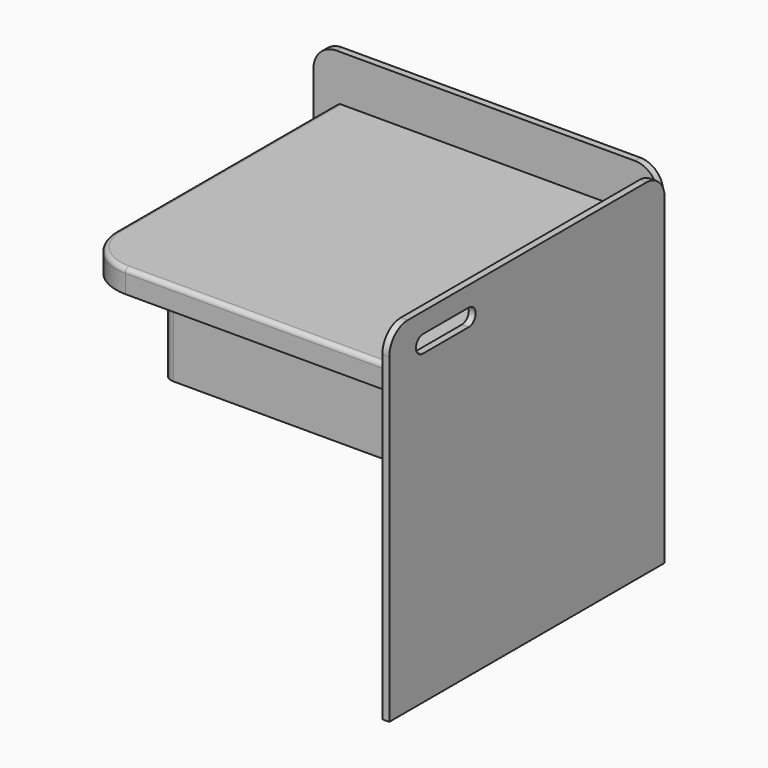
from build123d import *

# Parameters (mm, degrees)
F0_W      = 38.1
F0_H      = 38.1
F2_DEPTH  = 0.762
F1_W      = 38.1
F1_H      = 38.1
F3_DEPTH  = 0.762
F4_W      = 35.56
F4_H      = 35.56
F5_DEPTH  = 17.78
F8_W      = 30.48
F8_H      = 30.48
F9_DEPTH  = 10.16
F7_W      = 35.56
F7_H      = 35.56
F10_DEPTH = 2.54
F11_W     = 30.48
F11_H     = 12.7
F12_DEPTH = 1.27
F13_R     = 1.27
F14_DEPTH = 1.27
F16_R     = 1.27
F17_DEPTH = 2.54
F15_W     = 25.4
F15_H     = 7.62
F18_DEPTH = 1.27
F19_R     = 2.54
F19_2_R   = 2.54
F20_R     = 5.08
F21_R     = 1.27
F21_2_R   = 1.27
F23_DEPTH = 12.7
F24_DEPTH = 0.762
F26_W     = 38.1
F26_H     = 38.1
F27_DEPTH = 0.762
F29_DEPTH = 12.7
F30_R     = 2.54
F30_2_R   = 2.54
F31_T     = 1.27
F33_DEPTH = 25.4
F34_R     = 0.508
F35_R     = 0.508
F36_R     = 0.508
F37_R     = 2.54
F38_R     = 1.27


# Not quite as in the source:
# - a shell that OpenCascade refuses in one call is made with other operations: the cavity is built on its own and cut out
# - a feature names something its author has since deleted; it is built from what else it names


with BuildPart() as f2:
    # F0 (on Right) → F2 (new body)
    with BuildSketch(Plane.YZ):
        with Locations((-19.05, 19.05)):
            Rectangle(F0_W, F0_H)
    extrude(amount=-F2_DEPTH)

    # F19
    f19_edges = [f2.edges().sort_by_distance(p)[0] for p in [
        (-0.381, -38.1, 38.1),
        (-0.381, 0, 38.1),
    ]]
    fillet(f19_edges, radius=F19_R)

    # F22 (on face) → F23 (cut)
    with BuildSketch(Plane.YZ):
        with BuildLine():
            ThreePointArc((35.283215344, 34.4806989491), (34.330715344, 35.4331989491), (33.378215344, 34.4806989491))
            Line((33.378215344, 34.4806989491), (33.378215344, 28.1306989491))
            ThreePointArc((33.378215344, 28.1306989491), (34.330715344, 27.1781989491), (35.283215344, 28.1306989491))
            Line((35.283215344, 28.1306989491), (35.283215344, 34.4806989491))
        make_face()
    extrude(amount=-F23_DEPTH, mode=Mode.SUBTRACT)

    # F32 (on face) → F33 (cut)
    with BuildSketch(Plane(origin=(-0.762, 0, 0), x_dir=(0, -1, 0), z_dir=(-1, 0, 0))):
        with BuildLine():
            ThreePointArc((35.2714537645, 33.5571871057), (34.3189537645, 34.5096871057), (33.3664537645, 33.5571871057))
            Line((33.3664537645, 33.5571871057), (33.3664537645, 27.2071871057))
            ThreePointArc((33.3664537645, 27.2071871057), (34.3189537645, 26.2546871057), (35.2714537645, 27.2071871057))
            Line((35.2714537645, 27.2071871057), (35.2714537645, 33.5571871057))
        make_face()
    extrude(amount=-F33_DEPTH, mode=Mode.SUBTRACT)


with BuildPart() as f3:
    # F1 (on Front) → F3 (new body)
    with BuildSketch(Plane.XZ):
        with Locations((19.05, 19.05)):
            Rectangle(F1_W, F1_H)
    extrude(amount=F3_DEPTH)

    # F19#2
    f19_2_edges = [f3.edges().sort_by_distance(p)[0] for p in [
        (0, -0.381, 38.1),
    ]]
    fillet(f19_2_edges, radius=F19_2_R)


with BuildPart() as f5:
    # F4 (on Top) → F5 (new body)
    with BuildSketch(Plane.XY):
        with Locations((17.78, -18.5785688174)):
            Rectangle(F4_W, F4_H)
    extrude(amount=F5_DEPTH)

    # F21
    f21_edges = [f5.edges().sort_by_distance(p)[0] for p in [
        (35.56, -18.578569, 17.78),
    ]]
    fillet(f21_edges, radius=F21_R)


with BuildPart() as f9:
    # F8 (on offset) → F9 (new body)
    with BuildSketch(Plane.XY.offset(30.48)):
        with Locations((60.96, -16.002)):
            Rectangle(F8_W, F8_H)
    extrude(amount=-F9_DEPTH)

    # F21#2
    f21_2_edges = [f9.edges().sort_by_distance(p)[0] for p in [
        (45.72, -31.242, 25.4),
    ]]
    fillet(f21_2_edges, radius=F21_2_R)

    # F31: shell of thickness 1.27, made by hand


with BuildPart() as f10:
    # F7 (on offset) → F10 (new body)
    with BuildSketch(Plane.XY.offset(30.48)):
        with Locations((58.42, -18.542)):
            Rectangle(F7_W, F7_H)
    extrude(amount=F10_DEPTH)

    # F20
    f20_edges = [f10.edges().sort_by_distance(p)[0] for p in [
        (40.64, -36.322, 31.75),
    ]]
    fillet(f20_edges, radius=F20_R)

    # F34
    f34_edges = [f10.edges().sort_by_distance(p)[0] for p in [
        (40.64, -16.002, 33.02),
    ]]
    fillet(f34_edges, radius=F34_R)


with BuildPart() as f12:
    # F11 (on face) → F12 (new body)
    with BuildSketch(Plane.XZ.offset(36.3585688174)):
        with Locations((18.542, 8.89)):
            Rectangle(F11_W, F11_H)
    extrude(amount=F12_DEPTH)

    # F37
    f37_edges = [f12.edges().sort_by_distance(p)[0] for p in [
        (3.302, -36.993569, 15.24),
        (3.302, -36.993569, 2.54),
        (33.782, -36.993569, 2.54),
        (33.782, -36.993569, 15.24),
    ]]
    fillet(f37_edges, radius=F37_R)


with BuildPart() as f14:
    # F13 (on face) → F14 (new body)
    with BuildSketch(Plane.XZ.offset(37.6285688174)):
        with Locations((18.542, 8.89)):
            Circle(F13_R)
    extrude(amount=F14_DEPTH)

    # F35
    f35_edges = [f14.edges().sort_by_distance(p)[0] for p in [
        (17.272, -38.898569, 8.89),
    ]]
    fillet(f35_edges, radius=F35_R)


with BuildPart() as f17:
    # F16 (on face) → F17 (new body)
    with BuildSketch(Plane(origin=(45.72, 0, 0), x_dir=(0, -1, 0), z_dir=(-1, 0, 0))):
        with Locations((16.002, 25.4)):
            Circle(F16_R)
    extrude(amount=F17_DEPTH)

    # F36
    f36_edges = [f17.edges().sort_by_distance(p)[0] for p in [
        (43.18, -14.732, 25.4),
    ]]
    fillet(f36_edges, radius=F36_R)


with BuildPart() as f18:
    # F15 (on face) → F18 (new body)
    with BuildSketch(Plane(origin=(45.72, 0, 0), x_dir=(0, -1, 0), z_dir=(-1, 0, 0))):
        with Locations((16.002, 25.4)):
            Rectangle(F15_W, F15_H)
    extrude(amount=F18_DEPTH)

    # F38
    f38_edges = [f18.edges().sort_by_distance(p)[0] for p in [
        (45.085, -28.702, 21.59),
        (45.085, -28.702, 29.21),
        (45.085, -3.302, 21.59),
        (45.085, -3.302, 29.21),
    ]]
    fillet(f38_edges, radius=F38_R)


with BuildPart() as f24:
    # F1 (on Front) → F24 (new body)
    with BuildSketch(Plane.XZ):
        with Locations((57.15, 19.05)):
            Rectangle(F1_W, F1_H)
    extrude(amount=F24_DEPTH)

    # F30
    f30_edges = [f24.edges().sort_by_distance(p)[0] for p in [
        (76.2, -0.381, 38.1),
        (38.1, -0.381, 38.1),
    ]]
    fillet(f30_edges, radius=F30_R)


with BuildPart() as f27:
    # F26 (on offset) → F27 (new body)
    with BuildSketch(Plane.YZ.offset(76.2)):
        with Locations((-19.812, 19.05)):
            Rectangle(F26_W, F26_H)
    extrude(amount=F27_DEPTH)

    # F28 (on face) → F29 (cut)
    with BuildSketch(Plane.YZ.offset(76.962)):
        with BuildLine():
            Line((-27.8631728142, 35.8923991907), (-34.2131728142, 35.8923991907))
            ThreePointArc((-34.2131728142, 35.8923991907), (-35.1656728142, 34.9398991907), (-34.2131728142, 33.9873991907))
            Line((-34.2131728142, 33.9873991907), (-27.8631728142, 33.9873991907))
            ThreePointArc((-27.8631728142, 33.9873991907), (-26.9106728142, 34.9398991907), (-27.8631728142, 35.8923991907))
        make_face()
    extrude(amount=-F29_DEPTH, mode=Mode.SUBTRACT)

    # F30#2
    f30_2_edges = [f27.edges().sort_by_distance(p)[0] for p in [
        (76.581, -0.762, 38.1),
        (76.581, -38.862, 38.1),
    ]]
    fillet(f30_2_edges, radius=F30_2_R)


with BuildPart() as f31_core1:
    # F31_t2: copy of F9
    add(f9.part)

    # the walls: a layer under each face that stays
    f31_faces = [f31_core1.faces().sort_by_distance(p)[0] for p in [
        (45.72, -15.367, 25.4),
        (60.96, -16.002, 30.48),
        (60.96, -0.762, 25.4),
        (61.595, -31.242, 25.4),
        (76.2, -16.002, 25.4),
    ]]
    thicken(f31_faces, amount=-F31_T, mode=Mode.SUBTRACT)


with BuildPart() as f9_1:
    add(f9.part)

    # what is left inside the walls is the cavity
    f31_cavity = [f31_core1.part.solids().sort_by_distance(p)[0] for p in [
        (60.96, -20.658667, 20.3327),
    ]]
    add(f31_cavity, mode=Mode.SUBTRACT)


solid = Compound([f10.part, f17.part, f18.part, f24.part, f27.part, f9_1.part])
